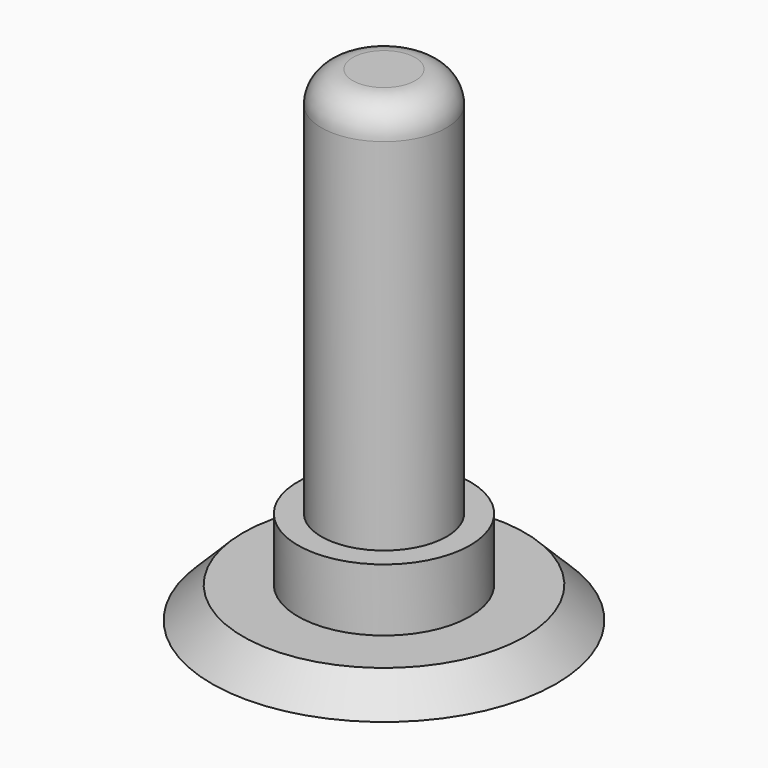
from build123d import *

# Parameters (mm, degrees)
F0_R     = 11
F1_DEPTH = 2
F2_R     = 5.5
F3_DEPTH = 4
F4_R     = 4
F5_DEPTH = 25
F6_R     = 2
F7_SIZE  = 1.99999
F8_T     = 2
F9_SIZE  = 3


# Not quite as in the source:
# - a fillet or chamfer is up to 0.001 mm smaller than in the source, because OpenCascade refuses the exact size
# - a shell that OpenCascade refuses in one call is made with other operations: the cavity is built on its own and cut out


with BuildPart() as f1:
    # F0 (on Top) → F1 (new body)
    with BuildSketch(Plane.XY):
        Circle(F0_R)
    extrude(amount=F1_DEPTH)

    # F2 (on face) → F3 (join)
    with BuildSketch(Plane.XY.offset(2)):
        Circle(F2_R)
    extrude(amount=F3_DEPTH)

    # F4 (on face) → F5 (join)
    with BuildSketch(Plane.XY.offset(6)):
        Circle(F4_R)
    extrude(amount=F5_DEPTH)

    # F6
    f6_edges = [f1.edges().sort_by_distance(p)[0] for p in [
        (-4, 0, 31),
    ]]
    fillet(f6_edges, radius=F6_R)

    # F7 (size 2 in the source; OpenCascade refuses exactly that, so slightly less here)
    f7_edges = [f1.edges().sort_by_distance(p)[0] for p in [
        (-11, 0, 2),
    ]]
    chamfer(f7_edges, length=F7_SIZE)

    # F8: shell of thickness 2, made by hand


with BuildPart() as f8_core1:
    # F8_t2: copy of F1
    add(f1.part)

    # the walls: a layer under each face that stays
    f8_faces = [f8_core1.faces().sort_by_distance(p)[0] for p in [
        (-6.0000066667, -6.0000066667, 2),
        (-10.000005, 0, 1.000005),
        (-5.5, 0, 4),
        (-11, 0, 5e-06),
        (-3.6666666667, -3.6666666667, 6),
        (-4, 0, 17.5),
        (0, 0, 31),
    ]]
    thicken(f8_faces, amount=-F8_T, mode=Mode.SUBTRACT)

    # F8_s3 → F8_t4 (revolve, cut)
    with BuildSketch(Plane.XZ):
        Polygon((5.52, 2.02), (5.5, 0), (3.5, 0), (3.5, 2), align=None)
    revolve(axis=Axis((0, 0, 2), (0, 0, 1)), mode=Mode.SUBTRACT)

    # F8_s5 → F8_t6 (revolve, cut)
    with BuildSketch(Plane.XZ):
        Polygon((4.02, 6.02), (4, 4), (2, 4), (2, 6), align=None)
    revolve(axis=Axis((0, 0, 6), (0, 0, 1)), mode=Mode.SUBTRACT)


with BuildPart() as f1_1:
    add(f1.part)

    # what is left inside the walls is the cavity
    f8_cavity = [f8_core1.part.solids().sort_by_distance(p)[0] for p in [
        (-1.98, 0, 12.333333),
    ]]
    add(f8_cavity, mode=Mode.SUBTRACT)

    # F9
    f9_edges = [f1_1.edges().sort_by_distance(p)[0] for p in [
        (-3.5, 0, 0),
    ]]
    chamfer(f9_edges, length=F9_SIZE)


solid = f1_1.part
